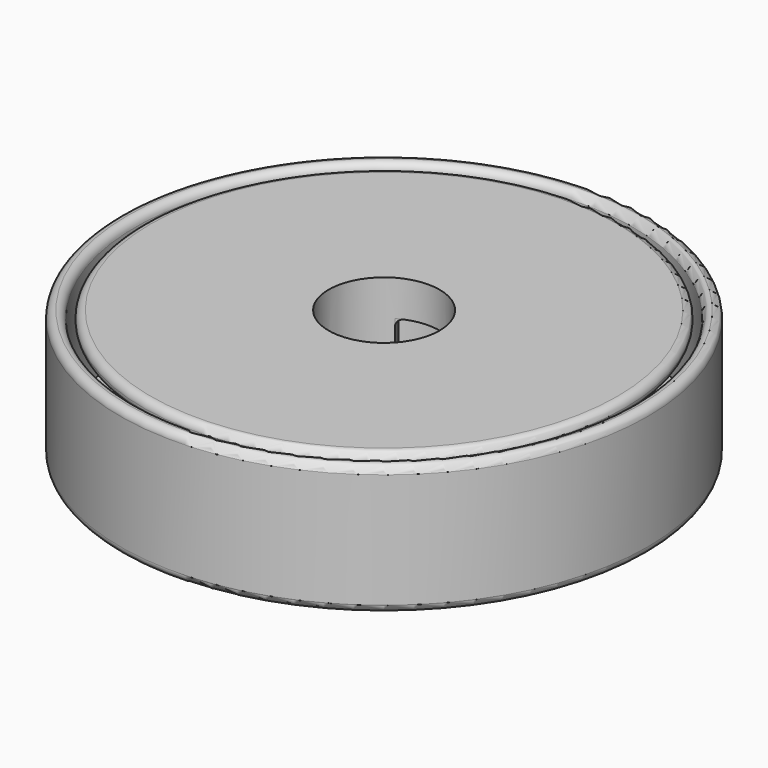
from build123d import *

# Parameters (mm, degrees)
F3_DEPTH     = 12.3
F4_T4_DEPTH  = 7.45
F4_S5_R      = 7.25
F4_T6_DEPTH  = 6
F4_S7_R      = 9.7
F4_T8_DEPTH  = 6
F4_T12_DEPTH = 7.45
F4_S13_R     = 7.25
F4_T14_DEPTH = 6
F4_S15_R     = 9.7
F4_T16_DEPTH = 6
F4_T20_DEPTH = 7.45
F4_S21_R     = 7.25
F4_T22_DEPTH = 5
F4_S23_R     = 9.7
F4_T24_DEPTH = 5
F4_T28_DEPTH = 7.45
F4_S29_R     = 7.25
F4_T30_DEPTH = 6
F4_S31_R     = 9.7
F4_T32_DEPTH = 6
F4_T36_DEPTH = 7.45
F4_S37_R     = 7.25
F4_T38_DEPTH = 6
F4_S39_R     = 9.7
F4_T40_DEPTH = 6
F4_T44_DEPTH = 7.45
F4_S45_R     = 7.25
F4_T46_DEPTH = 5
F4_S47_R     = 9.7
F4_T48_DEPTH = 5
F5_R         = 0.99999


# Not quite as in the source:
# - a fillet or chamfer that OpenCascade refuses, or shapes differently, is made with other operations: its cross-section is extruded or revolved along the edge and cut away or added
# - a fillet or chamfer is up to 0.001 mm smaller than in the source, because OpenCascade refuses the exact size


with BuildPart() as f1:
    # F0 (on Front) → F1 (revolve)
    with BuildSketch(Plane.XZ):
        Polygon((18.75, 12), (10, 12), (10, 3), (11.5, 3), (11.5, 0), (34.5, 0), (34.5, 17), (32.5, 17), (32.5, 2), (21.25, 2), (21.25, 4), (18.75, 4), align=None)
    revolve(axis=Axis((0, 0, 6), (0, 0, 1)))

    # F5 (radius 1 in the source; OpenCascade refuses exactly that, so slightly less here)
    f5_edges = [f1.edges().sort_by_distance(p)[0] for p in [
        (-32.5, 0, 17),
        (-34.5, 0, 17),
        (-34.5, 0, 0),
    ]]
    fillet(f5_edges, radius=F5_R)


with BuildPart() as f1b:
    # F0 (on Front) → F1, piece 2 (revolve)
    with BuildSketch(Plane.XZ):
        Polygon((31.5, 17), (7.25, 17), (7.25, 0), (9.4411542732, 0), (11, 2.7), (9.7, 2.7), (9.7, 12.3), (18.75, 12.3), (18.75, 15), (31.5, 15), align=None)
    revolve(axis=Axis((0, 0, 6), (0, 0, 1)))

    # F2 (on face) → F3 (cut, through all)
    with BuildSketch(Plane(origin=(0, 0, 0), x_dir=(1, 0, 0), z_dir=(0, 0, -1))):
        with BuildLine():
            Line((-4.7205771366, -8.1762794416), (-5.5, -9.5262794416))
            ThreePointArc((-5.5, -9.5262794416), (0, -11), (5.5, -9.5262794416))
            Line((5.5, -9.5262794416), (4.7205771366, -8.1762794416))
            ThreePointArc((4.7205771366, -8.1762794416), (0, -9.4411542732), (-4.7205771366, -8.1762794416))
        make_face()
        with BuildLine():
            Line((-3.625, -6.2786841774), (-4.7205771366, -8.1762794416))
            ThreePointArc((-4.7205771366, -8.1762794416), (0, -9.4411542732), (4.7205771366, -8.1762794416))
            Line((4.7205771366, -8.1762794416), (3.625, -6.2786841774))
            ThreePointArc((3.625, -6.2786841774), (0, -7.25), (-3.625, -6.2786841774))
        make_face()
        with BuildLine():
            Line((-11, 0), (-9.4411542732, 0))
            ThreePointArc((-9.4411542732, 0), (-8.1762794416, 4.7205771366), (-4.7205771366, 8.1762794416))
            Line((-4.7205771366, 8.1762794416), (-5.5, 9.5262794416))
            ThreePointArc((-5.5, 9.5262794416), (-9.5262794416, 5.5), (-11, 0))
        make_face()
        with BuildLine():
            Line((7.25, 0), (9.4411542732, 0))
            ThreePointArc((9.4411542732, 0), (8.1762794416, 4.7205771366), (4.7205771366, 8.1762794416))
            Line((4.7205771366, 8.1762794416), (3.625, 6.2786841774))
            ThreePointArc((3.625, 6.2786841774), (6.2786841774, 3.625), (7.25, 0))
        make_face()
        with BuildLine():
            ThreePointArc((4.7205771366, 8.1762794416), (8.1762794416, 4.7205771366), (9.4411542732, 0))
            Line((9.4411542732, 0), (11, 0))
            ThreePointArc((11, 0), (9.5262794416, 5.5), (5.5, 9.5262794416))
            Line((5.5, 9.5262794416), (4.7205771366, 8.1762794416))
        make_face()
        with BuildLine():
            ThreePointArc((-4.7205771366, 8.1762794416), (-8.1762794416, 4.7205771366), (-9.4411542732, 0))
            Line((-9.4411542732, 0), (-7.25, 0))
            ThreePointArc((-7.25, 0), (-6.2786841774, 3.625), (-3.625, 6.2786841774))
            Line((-3.625, 6.2786841774), (-4.7205771366, 8.1762794416))
        make_face()
    extrude(amount=-F3_DEPTH, mode=Mode.SUBTRACT)

    # F4: fillet of radius 1 on 8 edges, made by hand


with BuildPart() as f4_tool2:
    # F4_s3 → F4_t4 (new body)
    with BuildSketch(Plane(origin=(-2.375, 4.113620668, 0), x_dir=(0, 0, 1), z_dir=(-0.5, 0.8660254038, 0))):
        with BuildLine():
            ThreePointArc((12.3, 1), (12.0071067812, 0.2928932188), (11.3, 0))
            Line((11.3, 0), (12.3, 0))
            Line((12.3, 0), (12.3, 1))
        make_face()
    extrude(amount=F4_T4_DEPTH)

    # F4_s5 → F4_t6 (cut, symmetric)
    with BuildSketch(Plane.XY.offset(11.8)):
        Circle(F4_S5_R)
    extrude(amount=F4_T6_DEPTH, both=True, mode=Mode.SUBTRACT)

    # F4_s7 → F4_t8 (intersect, symmetric)
    with BuildSketch(Plane.XY.offset(11.8)):
        Circle(F4_S7_R)
    extrude(amount=F4_T8_DEPTH, both=True, mode=Mode.INTERSECT)


with BuildPart() as f1b_1:
    add(f1b.part)

    # F4_t1: union F4_tool2
    add(f4_tool2.part)


with BuildPart() as f4_tool10:
    # F4_s11 → F4_t12 (new body)
    with BuildSketch(Plane(origin=(6.1, 10.5655099262, 0), x_dir=(0, 0, 1), z_dir=(-0.5, -0.8660254038, 0))):
        with BuildLine():
            ThreePointArc((11.3, 0), (12.0071067812, 0.2928932188), (12.3, 1))
            Line((12.3, 1), (12.3, 0))
            Line((12.3, 0), (11.3, 0))
        make_face()
    extrude(amount=F4_T12_DEPTH)

    # F4_s13 → F4_t14 (cut, symmetric)
    with BuildSketch(Plane.XY.offset(11.8)):
        Circle(F4_S13_R)
    extrude(amount=F4_T14_DEPTH, both=True, mode=Mode.SUBTRACT)

    # F4_s15 → F4_t16 (intersect, symmetric)
    with BuildSketch(Plane.XY.offset(11.8)):
        Circle(F4_S15_R)
    extrude(amount=F4_T16_DEPTH, both=True, mode=Mode.INTERSECT)


with BuildPart() as f1b_2:
    add(f1b_1.part)

    # F4_t9: union F4_tool10
    add(f4_tool10.part)


with BuildPart() as f4_tool18:
    # F4_s19 → F4_t20 (new body)
    with BuildSketch(Plane.YZ.offset(-12.2)):
        with BuildLine():
            ThreePointArc((-1, 12.3), (-0.2928932188, 12.0071067812), (0, 11.3))
            Line((0, 11.3), (0, 12.3))
            Line((0, 12.3), (-1, 12.3))
        make_face()
    extrude(amount=F4_T20_DEPTH)

    # F4_s21 → F4_t22 (cut, symmetric)
    with BuildSketch(Plane.XY.offset(11.8)):
        Circle(F4_S21_R)
    extrude(amount=F4_T22_DEPTH, both=True, mode=Mode.SUBTRACT)

    # F4_s23 → F4_t24 (intersect, symmetric)
    with BuildSketch(Plane.XY.offset(11.8)):
        Circle(F4_S23_R)
    extrude(amount=F4_T24_DEPTH, both=True, mode=Mode.INTERSECT)


with BuildPart() as f1b_3:
    add(f1b_2.part)

    # F4_t17: union F4_tool18
    add(f4_tool18.part)


with BuildPart() as f4_tool26:
    # F4_s27 → F4_t28 (new body)
    with BuildSketch(Plane(origin=(-2.375, -4.113620668, 0), x_dir=(0, 0, 1), z_dir=(-0.5, -0.8660254038, 0))):
        with BuildLine():
            ThreePointArc((12.3, 1), (12.0071067812, 0.2928932188), (11.3, 0))
            Line((11.3, 0), (12.3, 0))
            Line((12.3, 0), (12.3, 1))
        make_face()
    extrude(amount=F4_T28_DEPTH)

    # F4_s29 → F4_t30 (cut, symmetric)
    with BuildSketch(Plane.XY.offset(11.8)):
        Circle(F4_S29_R)
    extrude(amount=F4_T30_DEPTH, both=True, mode=Mode.SUBTRACT)

    # F4_s31 → F4_t32 (intersect, symmetric)
    with BuildSketch(Plane.XY.offset(11.8)):
        Circle(F4_S31_R)
    extrude(amount=F4_T32_DEPTH, both=True, mode=Mode.INTERSECT)


with BuildPart() as f1b_4:
    add(f1b_3.part)

    # F4_t25: union F4_tool26
    add(f4_tool26.part)


with BuildPart() as f4_tool34:
    # F4_s35 → F4_t36 (new body)
    with BuildSketch(Plane(origin=(6.1, -10.5655099262, 0), x_dir=(0, 0, 1), z_dir=(-0.5, 0.8660254038, 0))):
        with BuildLine():
            ThreePointArc((12.3, 1), (12.0071067812, 0.2928932188), (11.3, 0))
            Line((11.3, 0), (12.3, 0))
            Line((12.3, 0), (12.3, 1))
        make_face()
    extrude(amount=F4_T36_DEPTH)

    # F4_s37 → F4_t38 (cut, symmetric)
    with BuildSketch(Plane.XY.offset(11.8)):
        Circle(F4_S37_R)
    extrude(amount=F4_T38_DEPTH, both=True, mode=Mode.SUBTRACT)

    # F4_s39 → F4_t40 (intersect, symmetric)
    with BuildSketch(Plane.XY.offset(11.8)):
        Circle(F4_S39_R)
    extrude(amount=F4_T40_DEPTH, both=True, mode=Mode.INTERSECT)


with BuildPart() as f1b_5:
    add(f1b_4.part)

    # F4_t33: union F4_tool34
    add(f4_tool34.part)


with BuildPart() as f4_tool42:
    # F4_s43 → F4_t44 (new body)
    with BuildSketch(Plane.YZ.offset(4.75)):
        with BuildLine():
            ThreePointArc((0, 11.3), (-0.2928932188, 12.0071067812), (-1, 12.3))
            Line((-1, 12.3), (0, 12.3))
            Line((0, 12.3), (0, 11.3))
        make_face()
    extrude(amount=F4_T44_DEPTH)

    # F4_s45 → F4_t46 (cut, symmetric)
    with BuildSketch(Plane.XY.offset(11.8)):
        Circle(F4_S45_R)
    extrude(amount=F4_T46_DEPTH, both=True, mode=Mode.SUBTRACT)

    # F4_s47 → F4_t48 (intersect, symmetric)
    with BuildSketch(Plane.XY.offset(11.8)):
        Circle(F4_S47_R)
    extrude(amount=F4_T48_DEPTH, both=True, mode=Mode.INTERSECT)


with BuildPart() as f1b_6:
    add(f1b_5.part)

    # F4_t41: union F4_tool42
    add(f4_tool42.part)

    # F4_s49 → F4_t50 (revolve, cut)
    with BuildSketch(Plane.XZ):
        with BuildLine():
            ThreePointArc((31.5, 16), (31.2071067812, 15.2928932188), (30.5, 15))
            Line((30.5, 15), (31.5, 15))
            Line((31.5, 15), (31.5, 16))
        make_face()
    revolve(axis=Axis((0, 0, 15), (0, 0, 1)), mode=Mode.SUBTRACT)

    # F4_s51 → F4_t52 (revolve, cut)
    with BuildSketch(Plane.XZ):
        with BuildLine():
            ThreePointArc((30.5, 17), (31.2071067812, 16.7071067812), (31.5, 16))
            Line((31.5, 16), (31.5, 17))
            Line((31.5, 17), (30.5, 17))
        make_face()
    revolve(axis=Axis((0, 0, 17), (0, 0, 1)), mode=Mode.SUBTRACT)


solid = Compound([f1.part, f1b_6.part])
